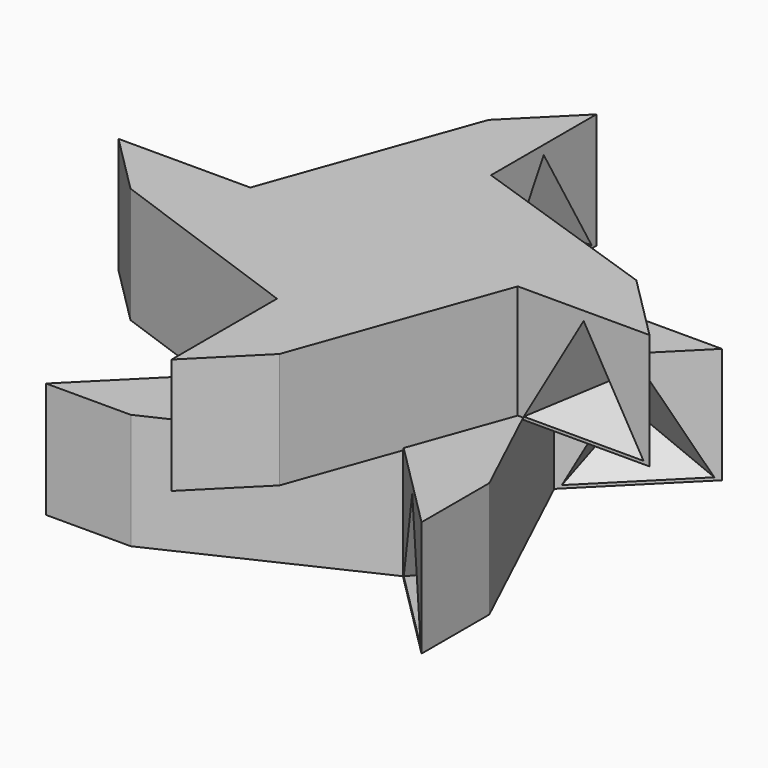
from build123d import *

# Parameters (mm, degrees)
F2_COUNT = 4
F4_DEPTH = 57.9615242271
F7_ANGLE = 45


# Not quite as in the source:
# - an extrude whose draft closes it to a point is written as a loft to that point


with BuildPart() as f1:
    # F0 (on Front) → F1 section 0
    with BuildSketch(Plane.XZ, mode=Mode.PRIVATE) as f1_s0:
        Polygon((70, 1.5), (130, 1.5), (100, 53.4615242271), align=None)
    loft([f1_s0.sketch, Vertex(100, 30, 18.8205080757)], ruled=True)


with BuildPart() as f2_1:
    # F2: instance of F1
    add(f1.part.rotate(Axis((0, 0, 19.4405535984), (0, 0, 1)), 1 * 360 / F2_COUNT))


with BuildPart() as f2_2:
    # F2: instance of F1
    add(f1.part.rotate(Axis((0, 0, 19.4405535984), (0, 0, 1)), 2 * 360 / F2_COUNT))


with BuildPart() as f2_3:
    # F2: instance of F1
    add(f1.part.rotate(Axis((0, 0, 19.4405535984), (0, 0, 1)), 3 * 360 / F2_COUNT))


with BuildPart() as f4:
    # F3 (on Top) → F4 (new body)
    with BuildSketch(Plane.XY):
        Polygon((67, 0), (133, 0), (100, 33), (0, 67), (0, 133), (-30, 103), (-67, 0), (-133, 0), (-103, -30), (0, -67), (0, -133), (30, -103), align=None)
    extrude(amount=F4_DEPTH)

    # F5: cut F1, F2_1, F2_2, F2_3
    add(f1.part, mode=Mode.SUBTRACT)
    add(f2_1.part, mode=Mode.SUBTRACT)
    add(f2_2.part, mode=Mode.SUBTRACT)
    add(f2_3.part, mode=Mode.SUBTRACT)


with BuildPart() as f6_1:
    # F6: copy of F4
    add(f4.part.moved(Location((0, 0, -57))))


with BuildPart() as f6_1_1:
    # F7: moved
    add(f6_1.part.rotate(Axis((0, 0, 19.4405535984), (0, 0, 1)), F7_ANGLE))


solid = Compound([f4.part, f6_1_1.part])
